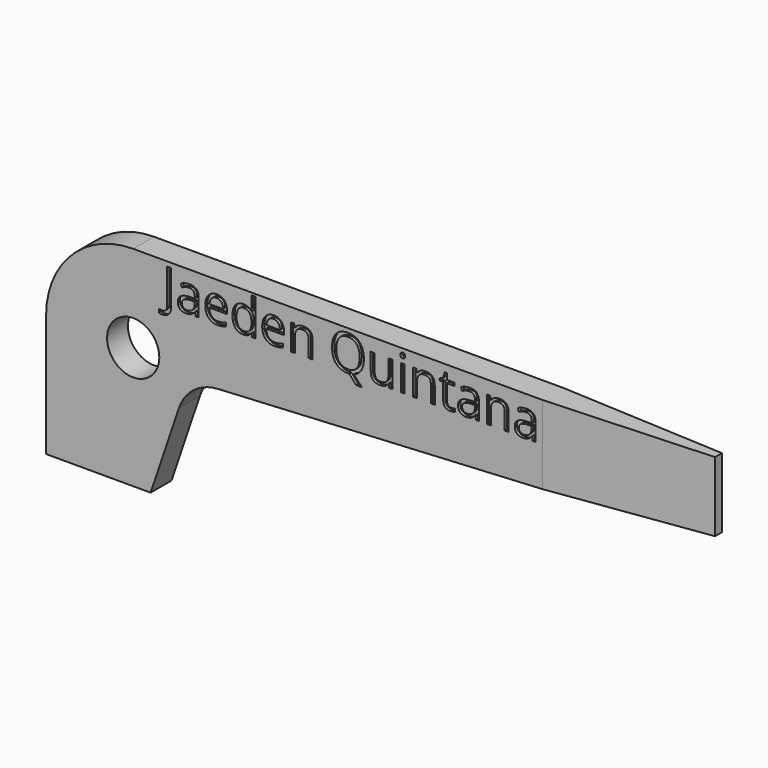
from build123d import *

# Parameters (mm, degrees)
F1_DEPTH     = 2.38125
F2_R         = 2.38125
F3_DEPTH     = 25.4
F5_DEPTH     = 25.4
F6_TEXT_SIZE = 4.4208946994
F7_DEPTH     = 0.254


# Not quite as in the source:
# - Text() gives the source's letters only with a copy of the font that has no kerning and outlines rounded to 1/6400 em; it was checked with that copy


with BuildPart() as f1:
    # F0 (on Front) → F1 (new body)
    with BuildSketch(Plane.XZ):
        with BuildLine():
            Line((60.325, 19.05), (7.9375, 19.05))
            ThreePointArc((7.9375, 19.05), (2.3248399243, 16.7251600757), (0, 11.1125))
            Line((0, 11.1125), (0, 0))
            Line((0, 0), (9.525, 0))
            Line((9.525, 0), (12.1103451907, 7.6262422093))
            ThreePointArc((12.1103451907, 7.6262422093), (13.4737562991, 9.5178776332), (15.6634210502, 10.3194652484))
            Line((15.6634210502, 10.3194652484), (60.325, 12.7))
            Line((60.325, 12.7), (60.325, 19.05))
        make_face()
    extrude(amount=F1_DEPTH)

    # F2 (on face) → F3 (cut)
    with BuildSketch(Plane.XZ.offset(2.38125)):
        with Locations((7.9375, 11.1125)):
            Circle(F2_R)
    extrude(amount=-F3_DEPTH, mode=Mode.SUBTRACT)

    # F4 (on face) → F5 (cut)
    with BuildSketch(Plane.XY.offset(19.05)):
        Polygon((60.325, -2.38125), (60.325, -1.5875), (45.24375, -2.38125), align=None)
        Polygon((60.325, 0), (45.24375, 0), (60.325, -0.79375), align=None)
    extrude(amount=-F5_DEPTH, mode=Mode.SUBTRACT)

    # F6 (on face) → F7 (cut)
    with BuildSketch(Plane.XZ.offset(2.38125)):
        with Locations((10.6198553258, 15.4730724309)):
            Text('Jaeden Quintana', F6_TEXT_SIZE, font='Open Sans', text_align=(TextAlign.LEFT, TextAlign.BOTTOM))
    extrude(amount=-F7_DEPTH, mode=Mode.SUBTRACT)


solid = f1.part
